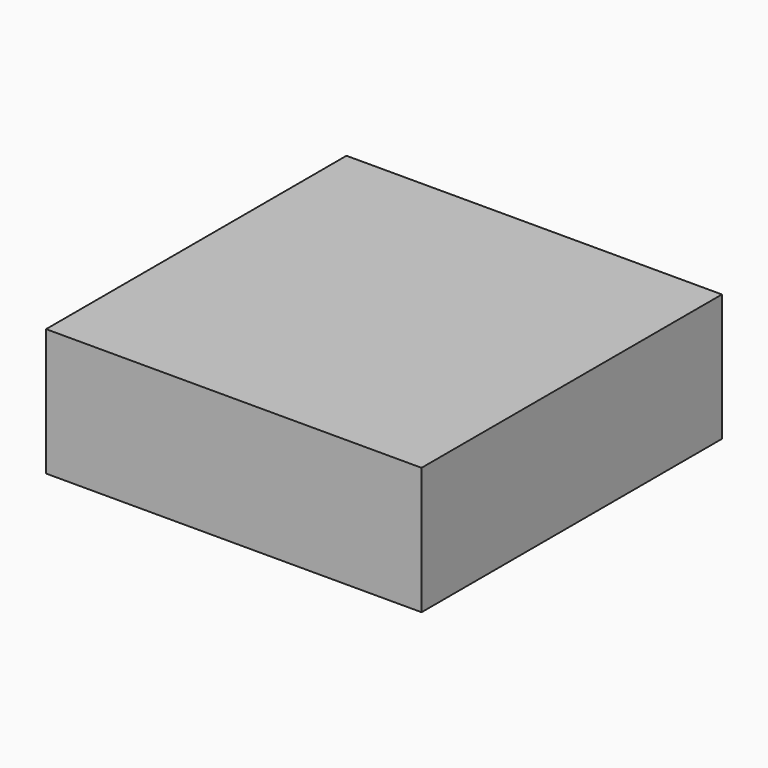
from build123d import *

# Parameters (mm, degrees)
F0_W     = 30
F0_H     = 30
F1_DEPTH = 10.16


with BuildPart() as f1:
    # F0 (on Top) → F1 (new body)
    with BuildSketch(Plane.XY):
        Rectangle(F0_W, F0_H)
    extrude(amount=F1_DEPTH)


solid = f1.part
